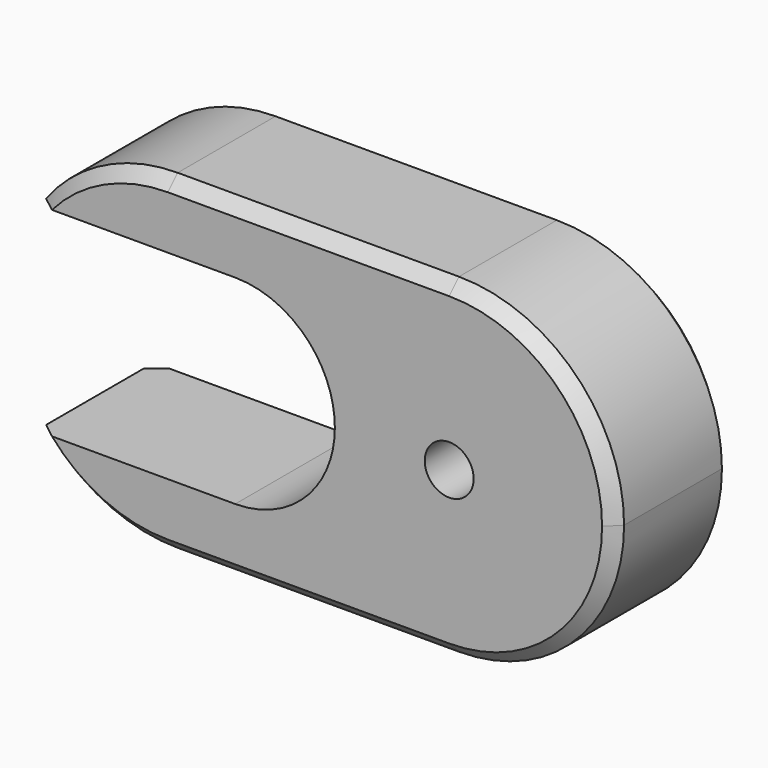
from build123d import *

# Parameters (mm, degrees)
F0_R     = 2
F1_DEPTH = 12
F2_SIZE  = 1


with BuildPart() as f1:
    # F0 (on Front) → F1 (new body)
    with BuildSketch(Plane.XZ):
        with BuildLine():
            ThreePointArc((-9.5, -13.5), (-2.9124896759, -11.7836627468), (2, -7.0710678119))
            ThreePointArc((2, -7.0710678119), (1.7096518051, -6.5755371981), (1.4406428571, -6.0681055776))
            ThreePointArc((1.4406428571, -6.0681055776), (-1.087317427, -7.6117527698), (-4, -8.15))
            Line((-4, -8.15), (-20.2623185234, -8.15))
            ThreePointArc((-20.2623185234, -8.15), (-15.5093676872, -12.0887344251), (-9.5, -13.5))
        make_face()
        with BuildLine():
            Line((-9.5, -13.5), (13.5, -13.5))
            ThreePointArc((13.5, -13.5), (6.9124896759, -11.7836627468), (2, -7.0710678119))
            ThreePointArc((2, -7.0710678119), (-2.9124896759, -11.7836627468), (-9.5, -13.5))
        make_face()
        with BuildLine():
            ThreePointArc((1.4406428571, 6.0681055776), (1.7096518051, 6.5755371981), (2, 7.0710678119))
            ThreePointArc((2, 7.0710678119), (-2.9124896759, 11.7836627468), (-9.5, 13.5))
            ThreePointArc((-9.5, 13.5), (-15.5093676872, 12.0887344251), (-20.2623185234, 8.15))
            Line((-20.2623185234, 8.15), (-4, 8.15))
            ThreePointArc((-4, 8.15), (-1.087317427, 7.6117527698), (1.4406428571, 6.0681055776))
        make_face()
        with BuildLine():
            ThreePointArc((3.7797727273, 2.4285049541), (3.1054603873, 4.8324288328), (2, 7.0710678119))
            ThreePointArc((2, 7.0710678119), (1.7096518051, 6.5755371981), (1.4406428571, 6.0681055776))
            ThreePointArc((1.4406428571, 6.0681055776), (2.8561301206, 4.4063567456), (3.7797727273, 2.4285049541))
        make_face()
        with BuildLine():
            ThreePointArc((2, 7.0710678119), (6.9124896759, 11.7836627468), (13.5, 13.5))
            Line((13.5, 13.5), (-9.5, 13.5))
            ThreePointArc((-9.5, 13.5), (-2.9124896759, 11.7836627468), (2, 7.0710678119))
        make_face()
        with BuildLine():
            ThreePointArc((13.5, -13.5), (23.045941546, -9.545941546), (27, 0))
            ThreePointArc((27, 0), (23.045941546, 9.545941546), (13.5, 13.5))
            ThreePointArc((13.5, 13.5), (6.9124896759, 11.7836627468), (2, 7.0710678119))
            ThreePointArc((2, 7.0710678119), (3.1054603873, 4.8324288328), (3.7797727273, 2.4285049541))
            ThreePointArc((3.7797727273, 2.4285049541), (4.0569115586, 1.2282817822), (4.15, 0))
            ThreePointArc((4.15, 0), (4.0569115586, -1.2282817822), (3.7797727273, -2.4285049541))
            ThreePointArc((3.7797727273, -2.4285049541), (3.1054603873, -4.8324288328), (2, -7.0710678119))
            ThreePointArc((2, -7.0710678119), (6.9124896759, -11.7836627468), (13.5, -13.5))
        make_face()
        with Locations((13.5, 0)):
            Circle(F0_R, mode=Mode.SUBTRACT)
        with BuildLine():
            ThreePointArc((1.4406428571, -6.0681055776), (1.7096518051, -6.5755371981), (2, -7.0710678119))
            ThreePointArc((2, -7.0710678119), (3.1054603873, -4.8324288328), (3.7797727273, -2.4285049541))
            ThreePointArc((3.7797727273, -2.4285049541), (2.8561301206, -4.4063567456), (1.4406428571, -6.0681055776))
        make_face()
    extrude(amount=F1_DEPTH)

    # F2
    f2_edges = [f1.edges().sort_by_distance(p)[0] for p in [
        (27, -12, 0),
        (27, 0, 0),
        (-15.509368, 0, -12.088734),
        (-15.509368, -12, -12.088734),
        (2, 0, -13.5),
        (2, -12, -13.5),
        (2, 0, 13.5),
        (2, -12, 13.5),
        (-15.509368, 0, 12.088734),
        (-15.509368, -12, 12.088734),
    ]]
    chamfer(f2_edges, length=F2_SIZE)


solid = f1.part
